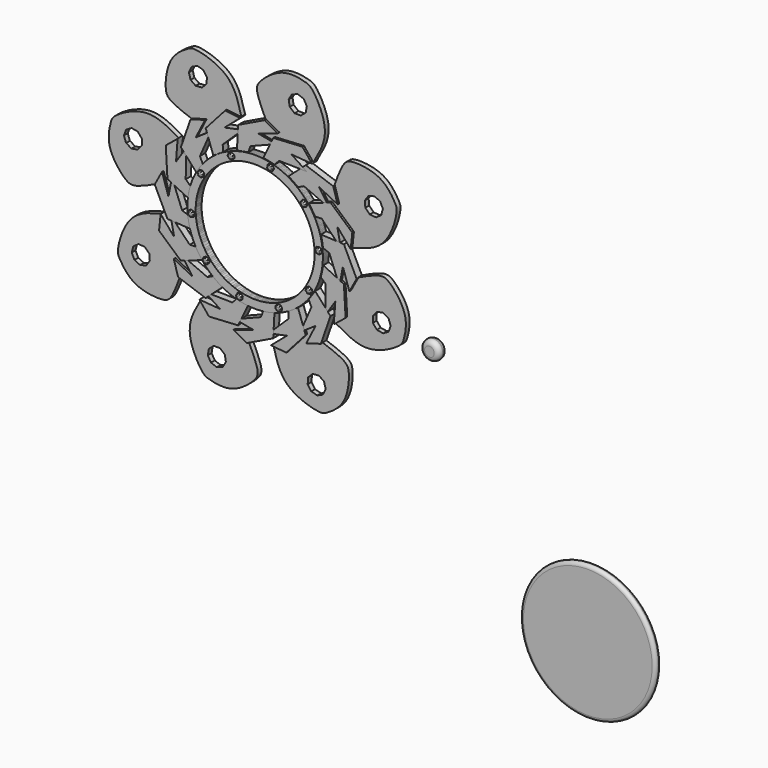
from build123d import *

# Parameters (mm, degrees)
F0_R          = 10
F1_DEPTH      = 1
F2_R          = 0.49999
F3_R          = 10
F4_DEPTH      = 1.1
F6_DEPTH      = 0.25
F6_DEPTH_BACK = 0.5
F7_T1_DEPTH   = 1.9107033262
F7_T3_DEPTH   = 1.9107033262
F7_T5_DEPTH   = 1.9107033262
F7_T7_DEPTH   = 1.9107033262
F7_T9_DEPTH   = 1.9107033262
F7_T11_DEPTH  = 1.9107033262
F7_T13_DEPTH  = 1.9107033262
F8_COUNT      = 10
F10_DEPTH     = 1
F11_COUNT     = 16
F13_DEPTH     = 0.7
F15_DEPTH     = 25
F16_COUNT     = 8
F17_R         = 1.4102589339
F18_DEPTH     = 1.5
F19_R         = 0.7


# Not quite as in the source:
# - a fillet or chamfer that OpenCascade refuses, or shapes differently, is made with other operations: its cross-section is extruded or revolved along the edge and cut away or added
# - a fillet or chamfer is up to 0.001 mm smaller than in the source, because OpenCascade refuses the exact size


with BuildPart() as f1:
    # F0 (on Front) → F1 (new body)
    with BuildSketch(Plane.XZ):
        Circle(F0_R)
    extrude(amount=F1_DEPTH)

    # F2 (radius 0.5 in the source; OpenCascade refuses exactly that, so slightly less here)
    f2_edges = [f1.edges().sort_by_distance(p)[0] for p in [
        (-10, -1, 0),
        (-10, 0, 0),
    ]]
    fillet(f2_edges, radius=F2_R)


with BuildPart() as f4:
    # F3 (on Front) → F4 (new body)
    with BuildSketch(Plane.XZ):
        with Locations((-49.048807472, 37.4402403831)):
            Circle(F3_R)
        with BuildLine():
            ThreePointArc((-40.2564157299, 37.6821715586), (-40.2539198776, 37.5612174143), (-40.2530878744, 37.4402403831))
            ThreePointArc((-40.2530878744, 37.4402403831), (-41.017097479, 33.8546696019), (-43.1764002162, 30.891995102))
            ThreePointArc((-43.1764002162, 30.891995102), (-43.8994673549, 30.3093933368), (-44.6799253208, 29.8062668445))
            ThreePointArc((-44.6799253208, 29.8062668445), (-48.622903267, 28.6548383521), (-52.6587688572, 29.4194634858))
            ThreePointArc((-52.6587688572, 29.4194634858), (-53.3236957566, 29.7532374955), (-53.9580364622, 30.1420108745))
            ThreePointArc((-53.9580364622, 30.1420108745), (-56.5061458809, 32.7762520582), (-57.7595091282, 36.2202568191))
            ThreePointArc((-57.7595091282, 36.2202568191), (-57.8412193703, 37.1990428499), (-57.8132926618, 38.1808364926))
            ThreePointArc((-57.8132926618, 38.1808364926), (-56.8327379462, 41.5359832476), (-54.6228376238, 44.2442738271))
            ThreePointArc((-54.6228376238, 44.2442738271), (-53.8873372615, 44.7855322572), (-53.0996819144, 45.2476150694))
            ThreePointArc((-53.0996819144, 45.2476150694), (-50.0311432035, 46.1809325611), (-46.8319854763, 45.952019485))
            ThreePointArc((-46.8319854763, 45.952019485), (-45.8168417491, 45.6206487352), (-44.849335857, 45.1687021573))
            ThreePointArc((-44.849335857, 45.1687021573), (-42.0736324457, 42.7985625638), (-40.4990444967, 39.5057273248))
            ThreePointArc((-40.4990444967, 39.5057273248), (-40.3299244318, 38.6003101101), (-40.2564157299, 37.6821715586))
        make_face(mode=Mode.SUBTRACT)
    extrude(amount=F4_DEPTH)

    # F5 (on face) → F6 (join, two sides)
    with BuildSketch(Plane.XZ.offset(1.1)) as f6_sk:
        Polygon((-57.9469229073, 36.784144579), (-58.1264023691, 37.1767482771), (-58.5452559144, 37.2812099854), (-58.8880782807, 37.0188679069), (-58.8967172337, 36.5872709775), (-58.5646674657, 36.311420488), (-58.1419692246, 36.3990374834), align=None)
    extrude(amount=F6_DEPTH)
    extrude(f6_sk.sketch, amount=-F6_DEPTH_BACK)

    # F7: fillet of radius 0.3 on 7 edges, made by hand

    # F7_s2 → F7_t1 (cut)
    with BuildSketch(Plane(origin=(2.4679452022, 0, 4.8728077635), x_dir=(0, 1, 0), z_dir=(0.451827256, 0, 0.8921054482))):
        with BuildLine():
            ThreePointArc((-1.1, 68.3148447424), (-1.2791287847, 68.4169995642), (-1.35, 68.6106487315))
            Line((-1.35, 68.6106487315), (-1.35, 68.3148447424))
            Line((-1.35, 68.3148447424), (-1.1, 68.3148447424))
        make_face()
    extrude(amount=F7_T1_DEPTH, mode=Mode.SUBTRACT)

    # F7_s4 → F7_t3 (cut)
    with BuildSketch(Plane(origin=(-23.6184457918, 0, 51.6643468272), x_dir=(0, 1, 0), z_dir=(-0.4157664388, 0, 0.9094714225))):
        with BuildLine():
            ThreePointArc((-1.1, 37.4074576123), (-1.2791287847, 37.5096124341), (-1.35, 37.7032616014))
            Line((-1.35, 37.7032616014), (-1.35, 37.4074576123))
            Line((-1.35, 37.4074576123), (-1.1, 37.4074576123))
        make_face()
    extrude(amount=F7_T3_DEPTH, mode=Mode.SUBTRACT)

    # F7_s6 → F7_t5 (cut)
    with BuildSketch(Plane(origin=(-62.7340367919, 0, 15.6458139663), x_dir=(0, 1, 0), z_dir=(-0.9702795251, 0, 0.2419868658))):
        with BuildLine():
            ThreePointArc((-1.1, -22.0060117303), (-1.2791287847, -21.9038569084), (-1.35, -21.7102077411))
            Line((-1.35, -21.7102077411), (-1.35, -22.0060117303))
            Line((-1.35, -22.0060117303), (-1.1, -22.0060117303))
        make_face()
    extrude(amount=F7_T5_DEPTH, mode=Mode.SUBTRACT)

    # F7_s8 → F7_t7 (cut)
    with BuildSketch(Plane(origin=(-18.3432132813, 0, -14.036997503), x_dir=(0, 1, 0), z_dir=(-0.7941523389, 0, -0.6077187365))):
        with BuildLine():
            ThreePointArc((-1.1, -65.1860090564), (-1.2791287847, -65.0838542345), (-1.35, -64.8902050672))
            Line((-1.35, -64.8902050672), (-1.35, -65.1860090564))
            Line((-1.35, -65.1860090564), (-1.1, -65.1860090564))
        make_face()
    extrude(amount=F7_T7_DEPTH, mode=Mode.SUBTRACT)

    # F7_s10 → F7_t9 (cut)
    with BuildSketch(Plane(origin=(0.7318974193, 0, 36.5651575303), x_dir=(0, 1, 0), z_dir=(-0.0200122438, 0, -0.999799735))):
        with BuildLine():
            ThreePointArc((-1.1, -59.6171156681), (-1.2791287847, -59.5149608462), (-1.35, -59.3213116789))
            Line((-1.35, -59.3213116789), (-1.35, -59.6171156681))
            Line((-1.35, -59.6171156681), (-1.1, -59.6171156681))
        make_face()
    extrude(amount=F7_T9_DEPTH, mode=Mode.SUBTRACT)

    # F7_s12 → F7_t11 (cut)
    with BuildSketch(Plane(origin=(-53.3995275063, 0, 44.3616807419), x_dir=(0, 1, 0), z_dir=(0.7691974791, 0, -0.6390111409))):
        with BuildLine():
            ThreePointArc((-1.1, -9.4928218715), (-1.2791287847, -9.3906670497), (-1.35, -9.1970178823))
            Line((-1.35, -9.1970178823), (-1.35, -9.4928218715))
            Line((-1.35, -9.4928218715), (-1.1, -9.4928218715))
        make_face()
    extrude(amount=F7_T11_DEPTH, mode=Mode.SUBTRACT)

    # F7_s14 → F7_t13 (cut)
    with BuildSketch(Plane(origin=(-49.6596259479, 0, -10.2934594775), x_dir=(0, 1, 0), z_dir=(0.9791858114, 0, 0.2029658758))):
        with BuildLine():
            ThreePointArc((-1.1, 47.4422567553), (-1.2791287847, 47.5444115771), (-1.35, 47.7380607444))
            Line((-1.35, 47.7380607444), (-1.35, 47.4422567553))
            Line((-1.35, 47.4422567553), (-1.1, 47.4422567553))
        make_face()
    extrude(amount=F7_T13_DEPTH, mode=Mode.SUBTRACT)


with BuildPart() as f8_1:
    # F8: instance of F4
    add(f4.part.rotate(Axis((-49.048807472, -1.1, 37.4402403831), (0, 1, 0)), 1 * 360 / F8_COUNT))


with BuildPart() as f8_2:
    # F8: instance of F4
    add(f4.part.rotate(Axis((-49.048807472, -1.1, 37.4402403831), (0, 1, 0)), 2 * 360 / F8_COUNT))


with BuildPart() as f8_3:
    # F8: instance of F4
    add(f4.part.rotate(Axis((-49.048807472, -1.1, 37.4402403831), (0, 1, 0)), 3 * 360 / F8_COUNT))


with BuildPart() as f8_4:
    # F8: instance of F4
    add(f4.part.rotate(Axis((-49.048807472, -1.1, 37.4402403831), (0, 1, 0)), 4 * 360 / F8_COUNT))


with BuildPart() as f8_5:
    # F8: instance of F4
    add(f4.part.rotate(Axis((-49.048807472, -1.1, 37.4402403831), (0, 1, 0)), 5 * 360 / F8_COUNT))


with BuildPart() as f8_6:
    # F8: instance of F4
    add(f4.part.rotate(Axis((-49.048807472, -1.1, 37.4402403831), (0, 1, 0)), 6 * 360 / F8_COUNT))


with BuildPart() as f8_7:
    # F8: instance of F4
    add(f4.part.rotate(Axis((-49.048807472, -1.1, 37.4402403831), (0, 1, 0)), 7 * 360 / F8_COUNT))


with BuildPart() as f8_8:
    # F8: instance of F4
    add(f4.part.rotate(Axis((-49.048807472, -1.1, 37.4402403831), (0, 1, 0)), 8 * 360 / F8_COUNT))


with BuildPart() as f8_9:
    # F8: instance of F4
    add(f4.part.rotate(Axis((-49.048807472, -1.1, 37.4402403831), (0, 1, 0)), 9 * 360 / F8_COUNT))


with BuildPart() as f10:
    # F9 (on Front) → F10 (new body)
    with BuildSketch(Plane.XZ):
        Polygon((-41.6625887156, 48.4837368131), (-44.182587415, 46.2272688746), (-42.7990555763, 45.2555045485), (-41.9096462429, 45.6672683358), (-38.1543524563, 44.0366826952), (-39.6861173213, 46.2931506336), (-36.9520001113, 44.9096225202), (-37.5943519175, 47.0672696829), align=None)
    extrude(amount=F10_DEPTH)


with BuildPart() as f11_1:
    # F11: instance of F10
    add(f10.part.rotate(Axis((-49.048807472, -1.1, 37.4402403831), (0, 1, 0)), 1 * 360 / F11_COUNT))


with BuildPart() as f11_2:
    # F11: instance of F10
    add(f10.part.rotate(Axis((-49.048807472, -1.1, 37.4402403831), (0, 1, 0)), 2 * 360 / F11_COUNT))


with BuildPart() as f11_3:
    # F11: instance of F10
    add(f10.part.rotate(Axis((-49.048807472, -1.1, 37.4402403831), (0, 1, 0)), 3 * 360 / F11_COUNT))


with BuildPart() as f11_4:
    # F11: instance of F10
    add(f10.part.rotate(Axis((-49.048807472, -1.1, 37.4402403831), (0, 1, 0)), 4 * 360 / F11_COUNT))


with BuildPart() as f11_5:
    # F11: instance of F10
    add(f10.part.rotate(Axis((-49.048807472, -1.1, 37.4402403831), (0, 1, 0)), 5 * 360 / F11_COUNT))


with BuildPart() as f11_6:
    # F11: instance of F10
    add(f10.part.rotate(Axis((-49.048807472, -1.1, 37.4402403831), (0, 1, 0)), 6 * 360 / F11_COUNT))


with BuildPart() as f11_7:
    # F11: instance of F10
    add(f10.part.rotate(Axis((-49.048807472, -1.1, 37.4402403831), (0, 1, 0)), 7 * 360 / F11_COUNT))


with BuildPart() as f11_8:
    # F11: instance of F10
    add(f10.part.rotate(Axis((-49.048807472, -1.1, 37.4402403831), (0, 1, 0)), 8 * 360 / F11_COUNT))


with BuildPart() as f11_9:
    # F11: instance of F10
    add(f10.part.rotate(Axis((-49.048807472, -1.1, 37.4402403831), (0, 1, 0)), 9 * 360 / F11_COUNT))


with BuildPart() as f11_10:
    # F11: instance of F10
    add(f10.part.rotate(Axis((-49.048807472, -1.1, 37.4402403831), (0, 1, 0)), 10 * 360 / F11_COUNT))


with BuildPart() as f11_11:
    # F11: instance of F10
    add(f10.part.rotate(Axis((-49.048807472, -1.1, 37.4402403831), (0, 1, 0)), 11 * 360 / F11_COUNT))


with BuildPart() as f11_12:
    # F11: instance of F10
    add(f10.part.rotate(Axis((-49.048807472, -1.1, 37.4402403831), (0, 1, 0)), 12 * 360 / F11_COUNT))


with BuildPart() as f11_13:
    # F11: instance of F10
    add(f10.part.rotate(Axis((-49.048807472, -1.1, 37.4402403831), (0, 1, 0)), 13 * 360 / F11_COUNT))


with BuildPart() as f11_14:
    # F11: instance of F10
    add(f10.part.rotate(Axis((-49.048807472, -1.1, 37.4402403831), (0, 1, 0)), 14 * 360 / F11_COUNT))


with BuildPart() as f11_15:
    # F11: instance of F10
    add(f10.part.rotate(Axis((-49.048807472, -1.1, 37.4402403831), (0, 1, 0)), 15 * 360 / F11_COUNT))


with BuildPart() as f13:
    # F12 (on Front) → F13 (new body)
    with BuildSketch(Plane.XZ):
        with BuildLine():
            Line((-61.1704848707, 44.7907522321), (-60.6593638659, 45.7278750837))
            add(Edge.make_bspline(
                [(-60.6593638659, 45.7278750837), (-62.2105684893, 46.6356149823), (-65.2736754723, 48.4280957292), (-70.2907225943, 45.6204343861), (-70.6995252166, 44.5847550564), (-71.4904502261, 41.1870058861), (-68.7496655724, 37.7614956693), (-67.2793774665, 37.0975582226), (-65.1865642396, 38.0884965716), (-63.892967999, 38.7010090053)],
                knots=[0, 0, 0, 0, 0.1829419886, 0.3612488478, 0.4449893544, 0.5880977892, 0.7514613793, 0.8463749076, 1, 1, 1, 1], degree=3))
            Line((-63.892967999, 38.7010090053), (-61.2190254033, 36.5245491266))
            Line((-61.2190254033, 36.5245491266), (-61.4504814148, 41.3978137076))
            Line((-61.4504814148, 41.3978137076), (-61.1704848707, 44.7907522321))
        make_face()
    extrude(amount=F13_DEPTH)

    # F14 (on face) → F15 (cut)
    with BuildSketch(Plane.XZ.offset(0.7)):
        Polygon((-66.1097988486, 42.9459910369), (-66.1097988486, 43.874469819), (-66.7066135056, 44.5857258306), (-67.6209866087, 44.7469544791), (-68.4250728209, 44.2827150881), (-68.742631267, 43.410230428), (-68.4250728209, 42.5377457679), (-67.6209866087, 42.0735063768), (-66.7066135056, 42.2347350254), align=None)
    extrude(amount=-F15_DEPTH, mode=Mode.SUBTRACT)


with BuildPart() as f16_1:
    # F16: instance of F13
    add(f13.part.rotate(Axis((-49.048807472, -1.1, 37.4402403831), (0, 1, 0)), 1 * 360 / F16_COUNT))


with BuildPart() as f16_2:
    # F16: instance of F13
    add(f13.part.rotate(Axis((-49.048807472, -1.1, 37.4402403831), (0, 1, 0)), 2 * 360 / F16_COUNT))


with BuildPart() as f16_3:
    # F16: instance of F13
    add(f13.part.rotate(Axis((-49.048807472, -1.1, 37.4402403831), (0, 1, 0)), 3 * 360 / F16_COUNT))


with BuildPart() as f16_4:
    # F16: instance of F13
    add(f13.part.rotate(Axis((-49.048807472, -1.1, 37.4402403831), (0, 1, 0)), 4 * 360 / F16_COUNT))


with BuildPart() as f16_5:
    # F16: instance of F13
    add(f13.part.rotate(Axis((-49.048807472, -1.1, 37.4402403831), (0, 1, 0)), 5 * 360 / F16_COUNT))


with BuildPart() as f16_6:
    # F16: instance of F13
    add(f13.part.rotate(Axis((-49.048807472, -1.1, 37.4402403831), (0, 1, 0)), 6 * 360 / F16_COUNT))


with BuildPart() as f16_7:
    # F16: instance of F13
    add(f13.part.rotate(Axis((-49.048807472, -1.1, 37.4402403831), (0, 1, 0)), 7 * 360 / F16_COUNT))


with BuildPart() as f18:
    # F17 (on Front) → F18 (new body)
    with BuildSketch(Plane.XZ):
        with Locations((-22.9902341962, 30.5183436722)):
            Circle(F17_R)
    extrude(amount=F18_DEPTH)

    # F19
    f19_edges = [f18.edges().sort_by_distance(p)[0] for p in [
        (-24.400493, -1.5, 30.518344),
        (-21.579975, -0.75, 30.518344),
        (-24.400493, 0, 30.518344),
    ]]
    fillet(f19_edges, radius=F19_R)


solid = Compound([f1.part, f4.part, f8_1.part, f8_2.part, f8_3.part, f8_4.part, f8_5.part, f8_6.part, f8_7.part, f8_8.part, f8_9.part, f10.part, f11_1.part, f11_2.part, f11_3.part, f11_4.part, f11_5.part, f11_6.part, f11_7.part, f11_8.part, f11_9.part, f11_10.part, f11_11.part, f11_12.part, f11_13.part, f11_14.part, f11_15.part, f13.part, f16_1.part, f16_2.part, f16_3.part, f16_4.part, f16_5.part, f16_6.part, f16_7.part, f18.part])
